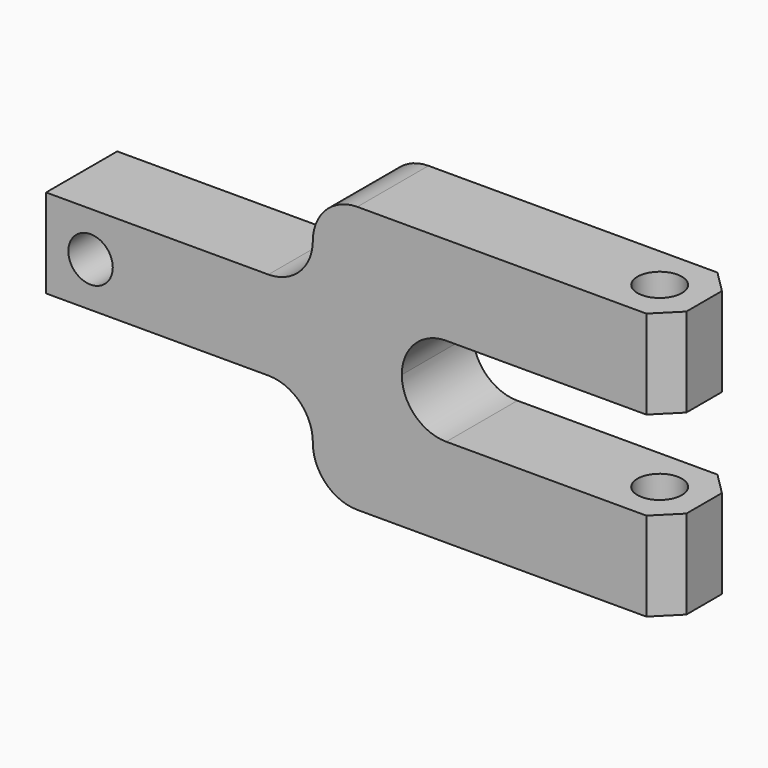
from build123d import *

# Parameters (mm, degrees)
F0_R     = 6.35
F1_DEPTH = 12.7
F2_R     = 6.35
F3_DEPTH = 44.45
F4_SIZE  = 6.35
F5_SIZE  = 6.35
F6_SIZE  = 6.35
F7_SIZE  = 6.35


# Not quite as in the source:
# - a feature names something its author has since deleted; it is built from what else it names


with BuildPart() as f1:
    # F0 (on Front) → F1 (new body, symmetric)
    with BuildSketch(Plane.XZ):
        with BuildLine():
            Line((-14.7091181397, 12.7), (-78.2091181397, 12.7))
            Line((-78.2091181397, 12.7), (-78.2091181397, -12.7))
            Line((-78.2091181397, -12.7), (-14.7091181397, -12.7))
            ThreePointArc((-14.7091181397, -12.7), (-5.7288620187, -16.4197438789), (-2.0091181397, -25.4))
            Line((-2.0091181397, -25.4), (-2.0091181397, -25.5123577416))
            ThreePointArc((-2.0091181397, -25.5123577416), (1.7106257392, -34.4926138626), (10.6908818603, -38.2123577416))
            Line((10.6908818603, -38.2123577416), (99.5908818603, -38.2123577416))
            Line((99.5908818603, -38.2123577416), (99.5908818603, -12.8123577416))
            Line((99.5908818603, -12.8123577416), (36.0908818603, -12.8123577416))
            ThreePointArc((36.0908818603, -12.8123577416), (27.1106257392, -9.0926138626), (23.3908818603, -0.1123577416))
            ThreePointArc((23.3908818603, -0.1123577416), (27.1106257392, 8.8678983795), (36.0908818603, 12.5876422584))
            Line((36.0908818603, 12.5876422584), (99.5908818603, 12.5876422584))
            Line((99.5908818603, 12.5876422584), (99.5908818603, 37.9876422584))
            Line((99.5908818603, 37.9876422584), (10.6908818603, 37.9876422584))
            ThreePointArc((10.6908818603, 37.9876422584), (1.7106257392, 34.2678983795), (-2.0091181397, 25.2876422584))
            Line((-2.0091181397, 25.2876422584), (-2.0091181397, 25.4))
            ThreePointArc((-2.0091181397, 25.4), (-5.7288620187, 16.4197438789), (-14.7091181397, 12.7))
        make_face()
        with Locations((-65.5091181397, 0)):
            Circle(F0_R, mode=Mode.SUBTRACT)
    extrude(amount=F1_DEPTH, both=True)

    # F2 (on Top) → F3 (cut, symmetric)
    with BuildSketch(Plane.XY):
        with Locations((86.8908818603, 0)):
            Circle(F2_R)
    extrude(amount=F3_DEPTH, both=True, mode=Mode.SUBTRACT)

    # F4
    f4_edges = [f1.edges().sort_by_distance(p)[0] for p in [
        (99.590882, -12.7, 25.287642),
    ]]
    chamfer(f4_edges, length=F4_SIZE)

    # F5
    f5_edges = [f1.edges().sort_by_distance(p)[0] for p in [
        (99.590882, 12.7, 25.287642),
    ]]
    chamfer(f5_edges, length=F5_SIZE)

    # F6
    f6_edges = [f1.edges().sort_by_distance(p)[0] for p in [
        (99.590882, -12.7, -25.512358),
    ]]
    chamfer(f6_edges, length=F6_SIZE)

    # F7
    f7_edges = [f1.edges().sort_by_distance(p)[0] for p in [
        (99.590882, 12.7, -25.512358),
    ]]
    chamfer(f7_edges, length=F7_SIZE)


solid = f1.part
